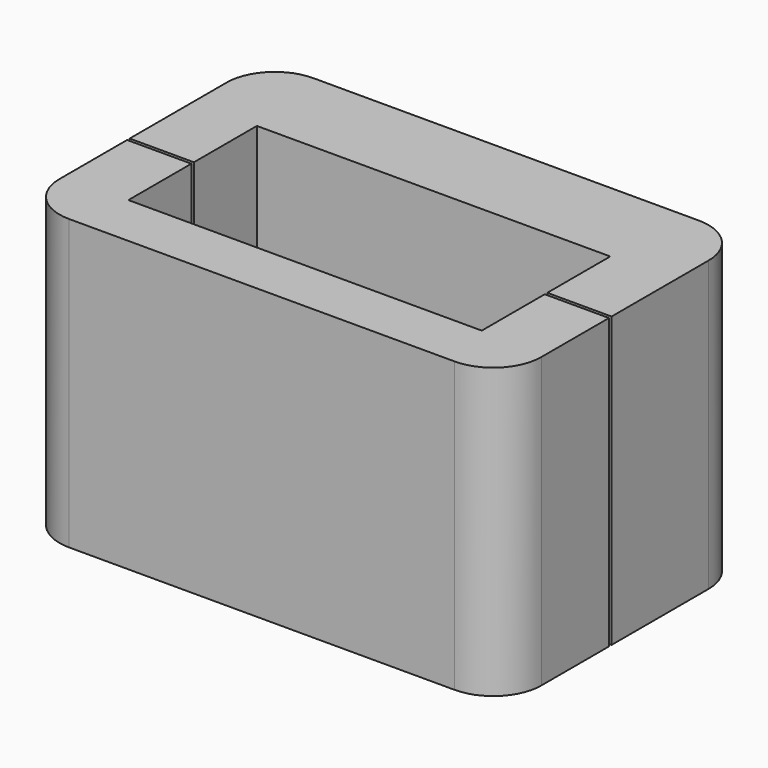
from build123d import *

# Parameters (mm, degrees)
F0_W     = 15
F0_H     = 9.5
F0_W_2   = 11
F0_H_2   = 5
F1_DEPTH = 9
F2_R     = 1.5
F0_R     = 2.25
F3_DEPTH = 1
F4_W     = 2
F4_H     = 0.1
F4_W_2   = 11
F5_DEPTH = 25


# Not quite as in the source:
# - a feature names something its author has since deleted; it is built from what else it names


with BuildPart() as f1:
    # F0 (on Top) → F1 (new body)
    with BuildSketch(Plane.XY):
        with Locations((0, 0.571324781)):
            Rectangle(F0_W, F0_H)
        Rectangle(F0_W_2, F0_H_2, mode=Mode.SUBTRACT)
    extrude(amount=F1_DEPTH)

    # F2
    f2_edges = [f1.edges().sort_by_distance(p)[0] for p in [
        (-7.5, 5.321325, 4.5),
        (7.5, 5.321325, 4.5),
        (7.5, -4.178675, 4.5),
        (-7.5, -4.178675, 4.5),
    ]]
    fillet(f2_edges, radius=F2_R)

    # F0 (on Top) → F3 (join)
    with BuildSketch(Plane.XY):
        Rectangle(F0_W_2, F0_H_2)
        Circle(F0_R, mode=Mode.SUBTRACT)
    extrude(amount=F3_DEPTH)

    # F4 (on face) → F5 (cut)
    with BuildSketch(Plane.XY.offset(9)):
        with Locations((-6.5, 0)):
            Rectangle(F4_W, F4_H)
        Rectangle(F4_W_2, F4_H)
        with Locations((6.5, 0)):
            Rectangle(F4_W, F4_H)
    extrude(amount=-F5_DEPTH, mode=Mode.SUBTRACT)


solid = f1.part
